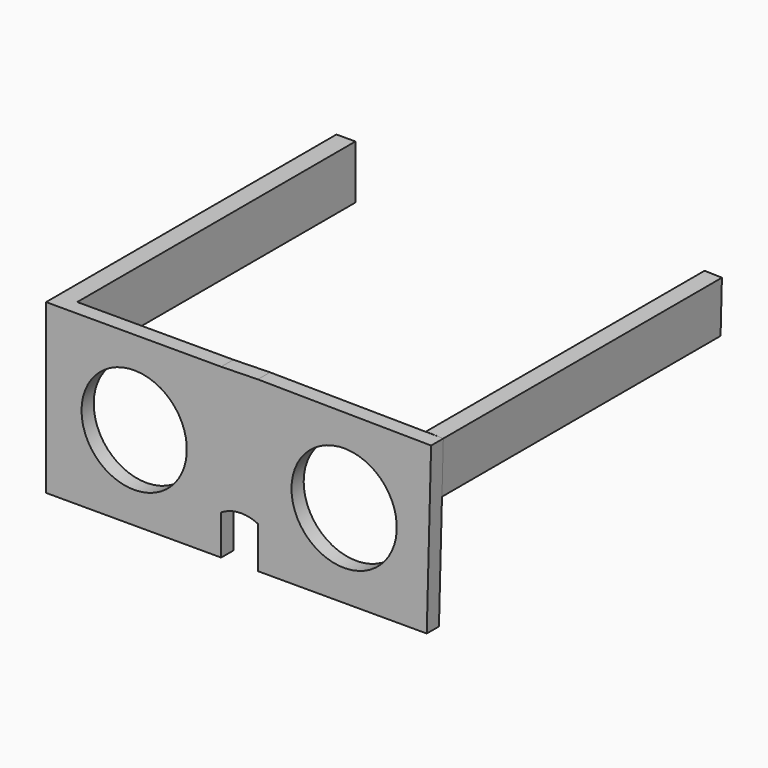
from build123d import *

# Parameters (mm, degrees)
F0_R     = 9.7397478584
F0_R_2   = 9.242675957
F1_DEPTH = 1.8415
F2_D     = 12.7
F4_W     = 41.9321846507
F4_H     = 6.4849769697
F5_DEPTH = 2.286
F3_W     = 41.9973064504
F3_H     = 6.2387038374
F6_DEPTH = 2.0955


# Not quite as in the source:
# - a feature names something its author has since deleted; it is built from what else it names


with BuildPart() as f1:
    # F0 (on Front) → F1 (new body)
    with BuildSketch(Plane.XZ):
        with BuildLine():
            Line((0, 4.8052047364), (0, 20.2608313411))
            Line((0, 20.2608313411), (-21.113075316, 20.2608313411))
            Line((-21.113075316, 20.2608313411), (-21.113075316, 0))
            Line((-21.113075316, 0), (-2.0606040489, 0))
            ThreePointArc((-2.0606040489, 0), (-1.7849391427, 2.7262115351), (0, 4.8052047364))
        make_face()
        with Locations((-10.4878218845, 10.1304156706)):
            Circle(F0_R, mode=Mode.SUBTRACT)
        with BuildLine():
            Line((25.3197303883, 20.1294401959), (4.4281314508, 20.3600343892))
            Line((4.4281314508, 20.3600343892), (4.4281314508, 19.6842234582))
            Line((4.4281314508, 19.6842234582), (4.4281314508, 5.0302978839))
            ThreePointArc((4.4281314508, 5.0302978839), (6.5221702803, 2.937211036), (6.8947323598, 0))
            Line((6.8947323598, 0), (24.7934444089, 0))
            Line((24.7934444089, 0), (25.3197303883, 20.1294401959))
        make_face()
        with Locations((14.8297464475, 10.0766858086)):
            Circle(F0_R_2, mode=Mode.SUBTRACT)
        with Locations((-10.4878218845, 10.1304156706)):
            Circle(F0_R)
        with Locations((14.8297464475, 10.0766858086)):
            Circle(F0_R_2)
        with BuildLine():
            Line((4.4281314508, 20.3600343892), (0, 20.2608313411))
            Line((0, 20.2608313411), (0, 4.8052047364))
            ThreePointArc((0, 4.8052047364), (2.1849540655, 5.490448695), (4.4281314508, 5.0302978839))
            Line((4.4281314508, 5.0302978839), (4.4281314508, 19.6842234582))
            Line((4.4281314508, 19.6842234582), (4.4281314508, 20.3600343892))
        make_face()
        with BuildLine():
            ThreePointArc((6.8947323598, 0), (6.5221702803, 2.937211036), (4.4281314508, 5.0302978839))
            Line((4.4281314508, 5.0302978839), (4.4281314508, 0))
            Line((4.4281314508, 0), (6.8947323598, 0))
        make_face()
        with BuildLine():
            Line((0, 0), (0, 4.8052047364))
            ThreePointArc((0, 4.8052047364), (-1.7849391427, 2.7262115351), (-2.0606040489, 0))
            Line((-2.0606040489, 0), (0, 0))
        make_face()
    extrude(amount=-F1_DEPTH)

    # F2 (through all)
    with Locations(Plane.XZ):
        with Locations((-10.4878218845, 10.1304156706), (14.8297464475, 10.0766858086)):
            Hole(F2_D / 2)

    # F4 (on face) → F5 (join)
    with BuildSketch(Plane(origin=(-21.113075316, 0, 0), x_dir=(0, -1, 0), z_dir=(-1, 0, 0))):
        with Locations((-22.8075923253, 17.0183428563)):
            Rectangle(F4_W, F4_H)
    extrude(amount=-F5_DEPTH)

    # F3 (on face) → F6 (join)
    with BuildSketch(Plane(origin=(24.77650804, 0, -0.6477839757), x_dir=(0, 1, 0), z_dir=(0.9996583923, 0, -0.0261361563))):
        with Locations((22.8401532252, 17.6649723378)):
            Rectangle(F3_W, F3_H)
    extrude(amount=-F6_DEPTH)


solid = f1.part
